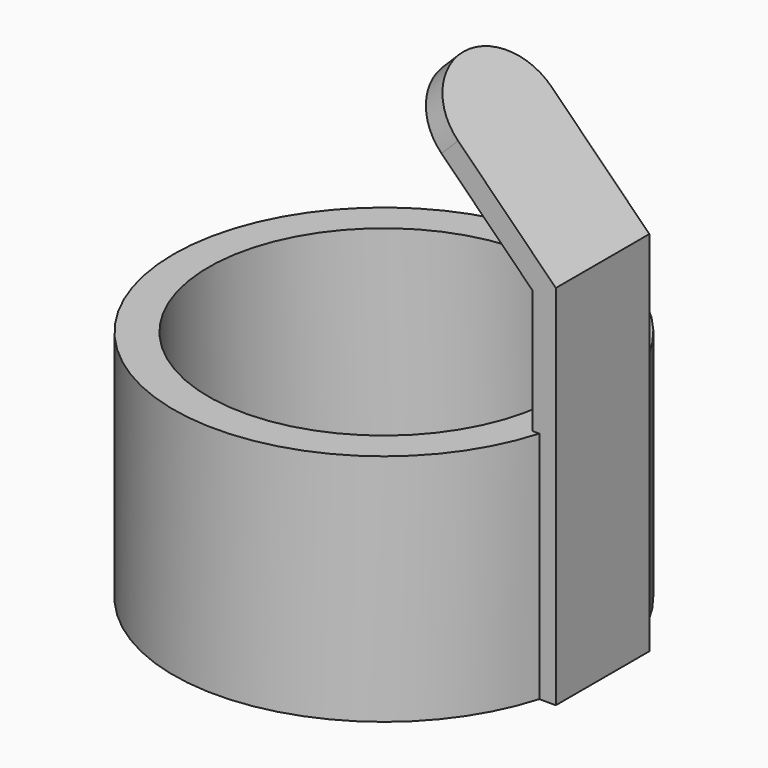
from build123d import *

# Parameters (mm, degrees)
F3_DEPTH = 25
F4_R     = 24.99999


# Not quite as in the source:
# - a fillet or chamfer is up to 0.001 mm smaller than in the source, because OpenCascade refuses the exact size


with BuildPart() as f1:
    # F0 (on Front) → F1 (revolve)
    with BuildSketch(Plane.XZ):
        Polygon((75, -25.5240468681), (0, -25.5240468681), (0, -40.5240468681), (90, -40.5240468681), (90, 59.4759531319), (75, 59.4759531319), align=None)
    revolve(axis=Axis((0, 0, -33.0240468681), (0, 0, -1)))

    # F2 (on Front) → F3 (join, symmetric)
    with BuildSketch(Plane.XZ):
        Polygon((83.5348658891, -40.5240468681), (93.5348658891, -40.5240468681), (93.5348658891, 116.5947673723), (34.0373912061, 176.0922420554), (26.9663233942, 169.0211742435), (83.5348658891, 112.4526317486), align=None)
    extrude(amount=F3_DEPTH, both=True)

    # F4 (radius 25 in the source; OpenCascade refuses exactly that, so slightly less here)
    f4_edges = [f1.edges().sort_by_distance(p)[0] for p in [
        (30.501857, -25, 172.556708),
        (30.501857, 25, 172.556708),
    ]]
    fillet(f4_edges, radius=F4_R)


solid = f1.part
